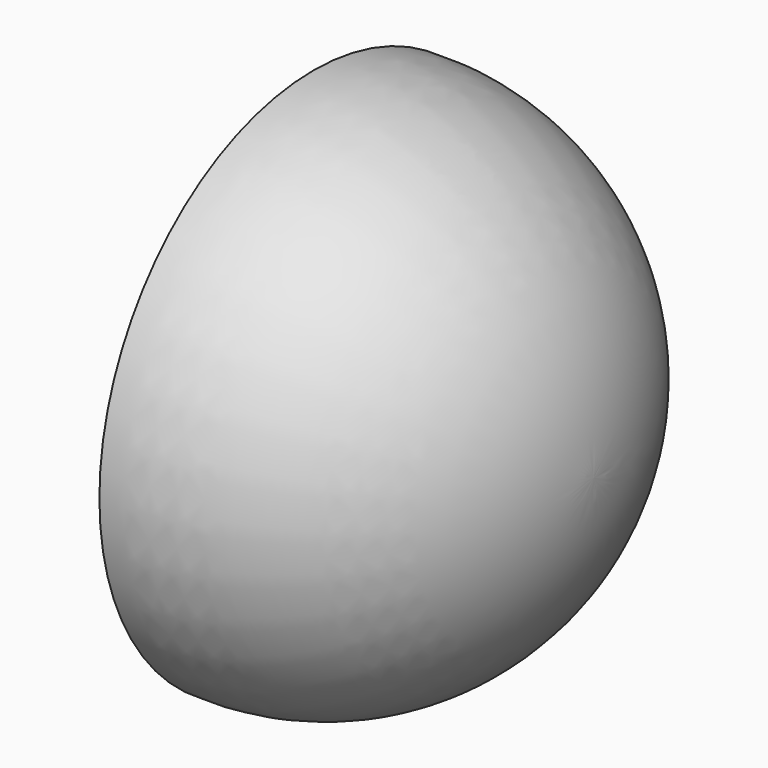
from build123d import *

# Parameters (mm, degrees)
F7_DEPTH  = 2.5
F13_DEPTH = 2
F25_DEPTH = 2
F30_R     = 0.6074168768
F31_DEPTH = 20
F32_R     = 1.25
F33_DEPTH = 25


# Not quite as in the source:
# - ends of sketch curves that miss each other by under 0.0002 mm in the source are joined
# - the program builds the solid bodies; features that only make, move or delete a surface that nothing else refers to are left out


with BuildPart() as f1:
    # F0 (on Front) → F1 (revolve)
    with BuildSketch(Plane.XZ):
        with BuildLine():
            Line((0, 20), (0, 0))
            Line((0, 0), (20.9032140208, 0))
            ThreePointArc((20.9032140208, 0), (14.7145025663, 14.4554109076), (0, 20))
        make_face()
    revolve(axis=Axis((10.4516070104, 0, 0), (1, 0, 0)))

    # F2 (on Right) → F3 (revolve)
    with BuildSketch(Plane.YZ):
        with BuildLine():
            Line((-3, 0), (0, 0))
            Line((0, 0), (0, 3))
            ThreePointArc((0, 3), (-2.1378188048, 2.1378188048), (-3, 0))
        make_face()
    revolve(axis=Axis((0, -1.5, 0), (0, -1, 0)))

    # F4 (on face) → F5 (revolve)
    with BuildSketch(Plane(origin=(0, 0, 0), x_dir=(0, -1, 0), z_dir=(-1, 0, 0))):
        with BuildLine():
            Line((-3, 0), (0, 0))
            Line((0, 0), (0, 3))
            ThreePointArc((0, 3), (-2.1060516761, 2.1060516761), (-3, 0))
        make_face()
    revolve(axis=Axis((0, 1.5, 0), (0, 1, 0)))

    # F20 (on face) → F21 (revolve)
    with BuildSketch(Plane(origin=(0, 0, 0), x_dir=(0, -1, 0), z_dir=(-1, 0, 0))):
        with BuildLine():
            ThreePointArc((-7.6594431885, -3.8764923811), (-8.2749807984, -4.5285373926), (-7.6594431885, -5.1805824041))
            Line((-7.6594431885, -5.1805824041), (-7.6594431885, -3.8764923811))
        make_face()
    revolve(axis=Axis((0, 7.6594431885, -4.5285373926), (0, 0, 1)))

    # F22 (on face) → F23 (revolve)
    with BuildSketch(Plane(origin=(0, 0, 0), x_dir=(0, -1, 0), z_dir=(-1, 0, 0))):
        with BuildLine():
            ThreePointArc((-5.9676826932, -12.5175017115), (-6.7753176022, -13.3251366206), (-5.9676826932, -14.1327715296))
            Line((-5.9676826932, -14.1327715296), (-5.9676826932, -12.5175017115))
        make_face()
    revolve(axis=Axis((0, 5.9676826932, -13.3251366206), (0, 0, 1)))

    # F28 (on face) → F29 (revolve)
    with BuildSketch(Plane(origin=(0, 0, 0), x_dir=(0, -1, 0), z_dir=(-1, 0, 0))):
        with BuildLine():
            ThreePointArc((2.2028738167, -10.7880309224), (1.6207013978, -10.2191004003), (1.0385289788, -10.7880309224))
            Line((1.0385289788, -10.7880309224), (2.2028738167, -10.7880309224))
        make_face()
    revolve(axis=Axis((0, -1.6207013978, -10.7880309224), (0, -1, 0)))

    # F30 (on face) → F31 (cut)
    with BuildSketch(Plane(origin=(0, 0, 0), x_dir=(0, -1, 0), z_dir=(-1, 0, 0))):
        with Locations((2.1903119247, -18.6780034797)):
            Circle(F30_R)
    extrude(amount=F31_DEPTH, mode=Mode.SUBTRACT)

    # F32 (on face) → F33 (cut)
    with BuildSketch(Plane(origin=(0, 0, 0), x_dir=(0, -1, 0), z_dir=(-1, 0, 0))):
        with Locations((-17.264097929, -2.2163949907)):
            Circle(F32_R)
    extrude(amount=-F33_DEPTH, mode=Mode.SUBTRACT)


with BuildPart() as f7:
    # F6 (on face) → F7 (new body)
    with BuildSketch(Plane(origin=(0, 0, 0), x_dir=(0, -1, 0), z_dir=(-1, 0, 0))):
        with BuildLine():
            add(Edge.make_bspline(
                [(13.0212418735, -3.58440727), (10.7913677509, -1.6396786361), (6.5594301058, -8.7429022088), (2.3274924606, -15.8461257815), (8.7893042283, -10.6876308427), (15.2511159961, -5.5291359038), (13.0212418735, -3.58440727)],
                knots=[0, 0, 0, 2.0943951024, 2.0943951024, 4.1887902048, 4.1887902048, 6.2831853072, 6.2831853072, 6.2831853072], degree=2, weights=[1, 0.5, 1, 0.5, 1, 0.5, 1]))
        make_face()
    extrude(amount=F7_DEPTH)


with BuildPart() as f13:
    # F12 (on face) → F13 (new body)
    with BuildSketch(Plane(origin=(0, 0, 0), x_dir=(0, -1, 0), z_dir=(-1, 0, 0))):
        with BuildLine():
            add(Edge.make_bspline(
                [(10.9271379188, 7.5598936528), (12.4094731309, 10.030454188), (5.7548497871, 12.3432447088), (-0.8997735567, 14.6560352296), (4.2725145749, 9.8726841736), (9.4448027066, 5.0893331176), (10.9271379188, 7.5598936528)],
                knots=[0, 0, 0, 2.0943951024, 2.0943951024, 4.1887902048, 4.1887902048, 6.2831853072, 6.2831853072, 6.2831853072], degree=2, weights=[1, 0.5, 1, 0.5, 1, 0.5, 1]))
        make_face()
    extrude(amount=F13_DEPTH)


with BuildPart() as f25:
    # F24 (on face) → F25 (new body)
    with BuildSketch(Plane(origin=(0, 0, 0), x_dir=(0, -1, 0), z_dir=(-1, 0, 0))):
        with BuildLine():
            add(Edge.make_bspline(
                [(-12.8653030843, -4.054680001), (-15.7865357239, -4.054680001), (-14.3259194041, -9.1504866723), (-12.8653030843, -14.2462933436), (-11.4046867644, -9.1504866723), (-9.9440704446, -4.054680001), (-12.8653030843, -4.054680001)],
                knots=[0, 0, 0, 2.0943951024, 2.0943951024, 4.1887902048, 4.1887902048, 6.2831853072, 6.2831853072, 6.2831853072], degree=2, weights=[1, 0.5, 1, 0.5, 1, 0.5, 1]))
        make_face()
    extrude(amount=F25_DEPTH)


solid = Compound([f1.part, f7.part, f13.part, f25.part])
